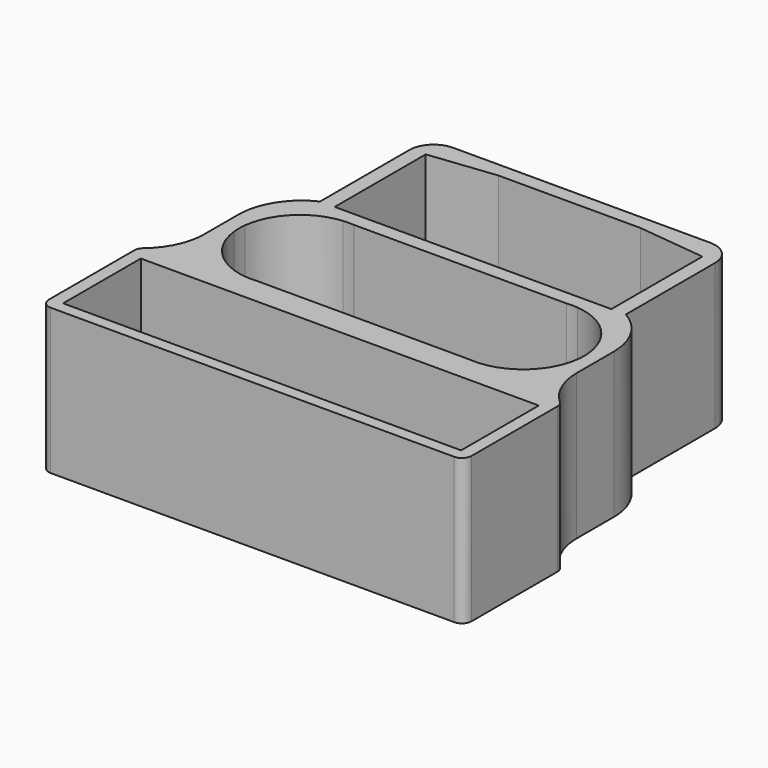
from build123d import *

# Parameters (mm, degrees)
F0_W        = 82
F0_H        = 20
F1_DEPTH    = 30
F2_T1_DEPTH = 30
F2_T3_DEPTH = 88.7163597955
F2_T5_DEPTH = 86.5103060247
F3_R        = 5
F4_R        = 2


# Not quite as in the source:
# - a fillet or chamfer that OpenCascade refuses, or shapes differently, is made with other operations: its cross-section is extruded or revolved along the edge and cut away or added


with BuildPart() as f1:
    # F0 (on Top) → F1 (new body)
    with BuildSketch(Plane.XY):
        Polygon((-31.3680246472, 15.4572909642), (-38.791685015, 15.4572909642), (-38.791685015, -15.5427090358), (38.208314985, -15.5427090358), (38.208314985, 15.4572909642), (31.6319753528, 15.4572909642), (28.6463200748, 15.4572909642), (-28.3536799252, 15.4572909642), align=None)
        with BuildLine():
            Line((-35.617634356, 1.409011777), (-35.617634356, 12.5002924819))
            Line((-35.617634356, 12.5002924819), (-24.2628612362, 12.5002924819))
            ThreePointArc((-24.2628612362, 12.5002924819), (-23.1469813734, 12.55), (-22.0311015107, 12.5002924819))
            Line((-22.0311015107, 12.5002924819), (21.7593006052, 12.5002924819))
            ThreePointArc((21.7593006052, 12.5002924819), (22.875180468, 12.55), (23.9910603307, 12.5002924819))
            Line((23.9910603307, 12.5002924819), (35.382365644, 12.5002924819))
            Line((35.382365644, 12.5002924819), (35.382365644, 1.035769749))
            ThreePointArc((35.382365644, 1.035769749), (35.4144721936, 0.5183271366), (35.425180468, 0))
            ThreePointArc((35.425180468, 0), (35.4144721936, -0.5183271366), (35.382365644, -1.035769749))
            Line((35.382365644, -1.035769749), (35.382365644, -12.4997075181))
            Line((35.382365644, -12.4997075181), (23.9975939216, -12.4997075181))
            ThreePointArc((23.9975939216, -12.4997075181), (22.875180468, -12.55), (21.7527670144, -12.4997075181))
            Line((21.7527670144, -12.4997075181), (-22.0245679198, -12.4997075181))
            ThreePointArc((-22.0245679198, -12.4997075181), (-23.1469813734, -12.55), (-24.269394827, -12.4997075181))
            Line((-24.269394827, -12.4997075181), (-35.617634356, -12.4997075181))
            Line((-35.617634356, -12.4997075181), (-35.617634356, -1.409011777))
            ThreePointArc((-35.617634356, -1.409011777), (-35.6969813734, 0), (-35.617634356, 1.409011777))
        make_face(mode=Mode.SUBTRACT)
        Polygon((38.208314985, -15.5427090358), (-38.791685015, -15.5427090358), (-44.0882174298, -15.5427090358), (-44.0882174298, -40.5095070601), (43.0414974689, -40.5095070601), (43.0414974689, -15.5427090358), align=None)
        with Locations((-0.4833955318, -28.0716251582)):
            Rectangle(F0_W, F0_H, mode=Mode.SUBTRACT)
        Polygon((-31.3680246472, 43.4572909642), (-31.3680246472, 15.4572909642), (-28.3536799252, 15.4572909642), (-28.3536799252, 38.9038845897), (-28.3536799252, 40.4572909642), (-14.6007314324, 40.4572909642), (14.6007314324, 40.4572909642), (28.6463200748, 40.4572909642), (28.6463200748, 38.9038845897), (28.6463200748, 15.4572909642), (31.6319753528, 15.4572909642), (31.6319753528, 43.4572909642), align=None)
        with BuildLine():
            Line((35.382365644, 12.5002924819), (23.9910603307, 12.5002924819))
            ThreePointArc((23.9910603307, 12.5002924819), (31.7777528847, 8.8457167242), (35.382365644, 1.035769749))
            Line((35.382365644, 1.035769749), (35.382365644, 12.5002924819))
        make_face()
        with BuildLine():
            ThreePointArc((35.382365644, -1.035769749), (31.7800643524, -8.8433897915), (23.9975939216, -12.4997075181))
            Line((23.9975939216, -12.4997075181), (35.382365644, -12.4997075181))
            Line((35.382365644, -12.4997075181), (35.382365644, -1.035769749))
        make_face()
        with BuildLine():
            Line((-24.2628612362, 12.5002924819), (-35.617634356, 12.5002924819))
            Line((-35.617634356, 12.5002924819), (-35.617634356, 1.409011777))
            ThreePointArc((-35.617634356, 1.409011777), (-31.9163938742, 8.9777449503), (-24.2628612362, 12.5002924819))
        make_face()
        with BuildLine():
            ThreePointArc((-24.269394827, -12.4997075181), (-31.9187398511, -8.9754528136), (-35.617634356, -1.409011777))
            Line((-35.617634356, -1.409011777), (-35.617634356, -12.4997075181))
            Line((-35.617634356, -12.4997075181), (-24.269394827, -12.4997075181))
        make_face()
        Polygon((14.6007314324, 40.4572909642), (28.6463200748, 38.9038845897), (28.6463200748, 40.4572909642), align=None)
        Polygon((-28.3536799252, 40.4572909642), (-28.3536799252, 38.9038845897), (-14.6007314324, 40.4572909642), align=None)
    extrude(amount=F1_DEPTH)

    # F2: fillet of radius 13 on 4 edges, made by hand

    # F2_s2 → F2_t1 (join)
    with BuildSketch(Plane.XY):
        with BuildLine():
            ThreePointArc((-38.791685015, -5.0710049164), (-40.1911445403, -10.9384967738), (-44.0882174298, -15.5427090358))
            Line((-44.0882174298, -15.5427090358), (-38.791685015, -15.5427090358))
            Line((-38.791685015, -15.5427090358), (-38.791685015, -5.0710049164))
        make_face()
        with BuildLine():
            ThreePointArc((43.0414974689, -15.5427090358), (39.4786809816, -11.0331797269), (38.208314985, -5.4282099548))
            Line((38.208314985, -5.4282099548), (38.208314985, -15.5427090358))
            Line((38.208314985, -15.5427090358), (43.0414974689, -15.5427090358))
        make_face()
    extrude(amount=F2_T1_DEPTH)

    # F2_s4 → F2_t3 (cut)
    with BuildSketch(Plane.XY.offset(-29.3581798978)):
        with BuildLine():
            ThreePointArc((-38.791685015, 3.7140190051), (-36.7801429418, 10.6605139767), (-31.3680246472, 15.4572909642))
            Line((-31.3680246472, 15.4572909642), (-38.791685015, 15.4572909642))
            Line((-38.791685015, 15.4572909642), (-38.791685015, 3.7140190051))
        make_face()
    extrude(amount=F2_T3_DEPTH, mode=Mode.SUBTRACT)

    # F2_s6 → F2_t5 (cut)
    with BuildSketch(Plane.XY.offset(-28.2551530123)):
        with BuildLine():
            ThreePointArc((38.208314985, 4.1552297593), (36.44458627, 10.6932881568), (31.6319753528, 15.4572909642))
            Line((31.6319753528, 15.4572909642), (38.208314985, 15.4572909642))
            Line((38.208314985, 15.4572909642), (38.208314985, 4.1552297593))
        make_face()
    extrude(amount=F2_T5_DEPTH, mode=Mode.SUBTRACT)

    # F3
    f3_edges = [f1.edges().sort_by_distance(p)[0] for p in [
        (31.631975, 43.457291, 15),
        (-31.368025, 43.457291, 15),
    ]]
    fillet(f3_edges, radius=F3_R)

    # F4
    f4_edges = [f1.edges().sort_by_distance(p)[0] for p in [
        (-44.088217, -15.542709, 15),
        (-44.088217, -40.509507, 15),
        (43.041497, -40.509507, 15),
        (43.041497, -15.542709, 15),
    ]]
    fillet(f4_edges, radius=F4_R)


solid = f1.part
